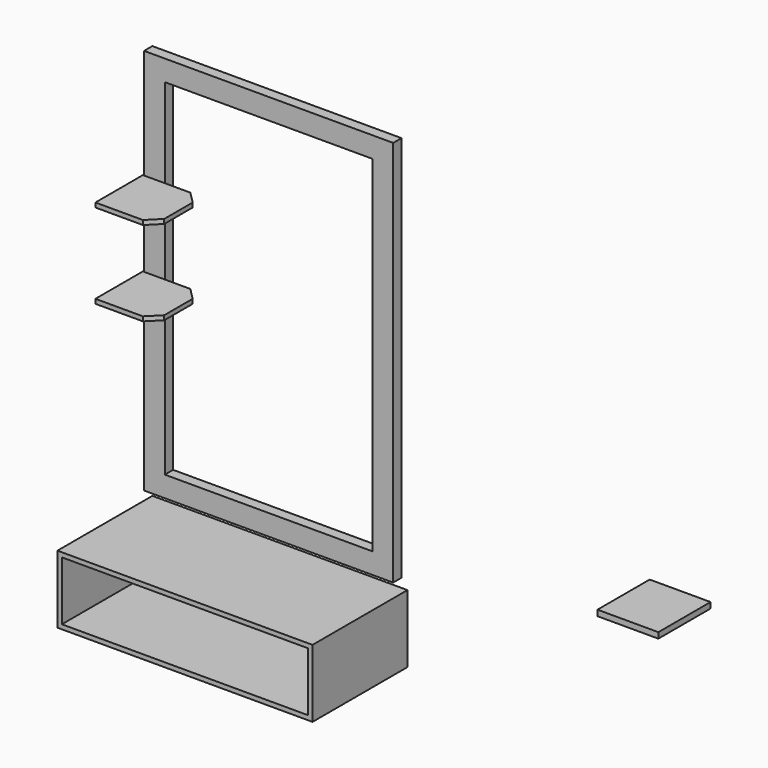
from build123d import *

# Parameters (mm, degrees)
F0_W      = 1092.2
F0_H      = 290.4416266203
F1_DEPTH  = 508
F6_START  = 330.2
F0_W_2    = 63.5
F0_H_2    = 24.6255362988
F0_W_3    = 197.2212322235
F6_DEPTH  = 279.4
F7_START  = 50.8
F0_W_4    = 88.9
F0_H_3    = 19.05
F0_W_5    = 165.1
F7_DEPTH  = 254
F8_SIZE   = 50.8
F8_2_SIZE = 50.8
F0_H_4    = 343.9922002792
F9_DEPTH  = 44.45
F10_T     = -19.05


# Not quite as in the source:
# - the program builds the solid bodies; features that only make, move or delete a surface that nothing else refers to are left out


with BuildPart() as f1:
    # F0 (on Front) → F1 (new body)
    with BuildSketch(Plane.XZ):
        with Locations((546.1, 311.9791866899)):
            Rectangle(F0_W, F0_H)
    extrude(amount=F1_DEPTH)

    # F10
    f10_openings = [f1.faces().sort_by_distance(p)[0] for p in [
        (546.1, -508, 311.979187),
    ]]
    offset(amount=F10_T, openings=f10_openings)


with BuildPart() as f6:
    # F0 (on Front) → F6 (new body)
    with BuildSketch(Plane.XZ.offset(F6_START)):
        with Locations((2622.55, 1042.1009046316)):
            Rectangle(F0_W_2, F0_H_2)
        with Locations((2492.1893838882, 1042.1009046316)):
            Rectangle(F0_W_3, F0_H_2)
    extrude(amount=F6_DEPTH)


with BuildPart() as f7:
    # F0 (on Front) → F7 (new body)
    with BuildSketch(Plane.XZ.offset(F7_START)):
        with Locations((44.45, 1677.4922002792)):
            Rectangle(F0_W_4, F0_H_3)
        with Locations((171.45, 1677.4922002792)):
            Rectangle(F0_W_5, F0_H_3)
    extrude(amount=F7_DEPTH)

    # F8
    f8_edges = [f7.edges().sort_by_distance(p)[0] for p in [
        (254, -304.8, 1677.4922),
        (254, -50.8, 1677.4922),
    ]]
    chamfer(f8_edges, length=F8_SIZE)


with BuildPart() as f7b:
    # F0 (on Front) → F7, piece 2 (new body)
    with BuildSketch(Plane.XZ.offset(F7_START)):
        with Locations((44.45, 1314.45)):
            Rectangle(F0_W_4, F0_H_3)
        with Locations((171.45, 1314.45)):
            Rectangle(F0_W_5, F0_H_3)
    extrude(amount=F7_DEPTH)

    # F8#2
    f8_2_edges = [f7b.edges().sort_by_distance(p)[0] for p in [
        (254, -304.8, 1314.45),
        (254, -50.8, 1314.45),
    ]]
    chamfer(f8_2_edges, length=F8_2_SIZE)


with BuildPart() as f9:
    # F0 (on Front) → F9 (new body)
    with BuildSketch(Plane.XZ):
        with Locations((44.45, 1314.45)):
            Rectangle(F0_W_4, F0_H_3)
        with Locations((44.45, 1495.9711001396)):
            Rectangle(F0_W_4, F0_H_4)
        with Locations((44.45, 1677.4922002792)):
            Rectangle(F0_W_4, F0_H_3)
        Polygon((0, 1304.925), (0, 495.3), (1066.8, 495.3), (1066.8, 2152.65), (0, 2152.65), (0, 1687.0172002792), (88.9, 1687.0172002792), (88.9, 2063.75), (977.9, 2063.75), (977.9, 584.2), (88.9, 584.2), (88.9, 1304.925), align=None)
    extrude(amount=F9_DEPTH)


solid = Compound([f1.part, f6.part, f7.part, f7b.part, f9.part])
